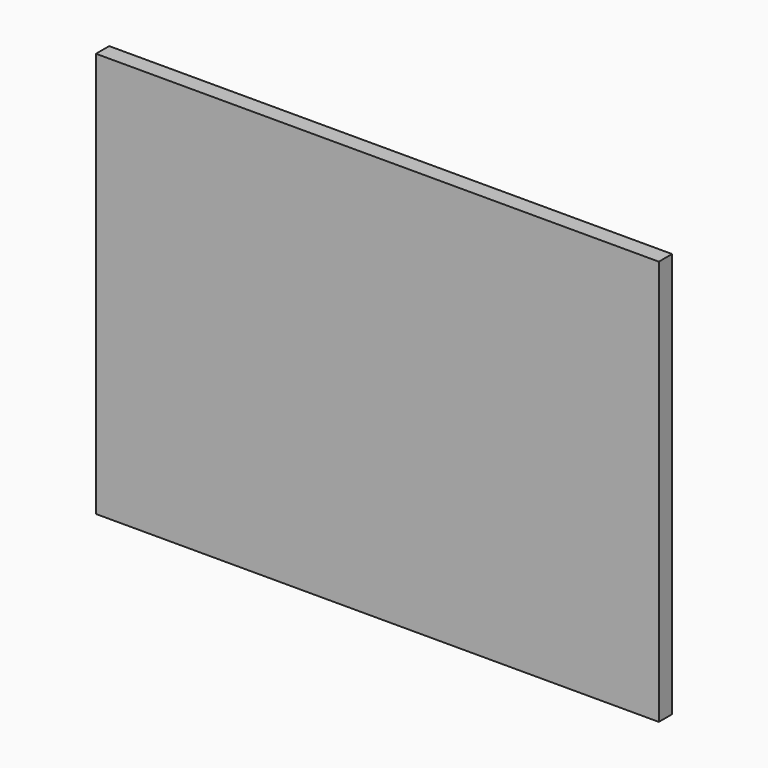
from build123d import *

# Parameters (mm, degrees)
F0_W     = 170
F0_H     = 122.3707973333
F1_DEPTH = 5
F2_R     = 1.5
F3_DEPTH = 5


# Not quite as in the source:
# - a pattern or mirror of a feature is missing from the dataset's text; its kind, count and spacing are read off the source's solid


with BuildPart() as f1:
    # F0 (on Front) → F1 (new body)
    with BuildSketch(Plane.XZ):
        Rectangle(F0_W, F0_H)
    extrude(amount=F1_DEPTH)

    # F2 (on Front) → F3 (join)
    with BuildSketch(Plane.XZ):
        with Locations((70, 56.1853986666)):
            Circle(F2_R)
    f3 = extrude(amount=-F3_DEPTH)

    # F3_copies: F3 across plane
    add(f3.mirror(Plane(origin=(0, 0, 0), x_dir=(0, 0, -1), z_dir=(-1, 0, 0))))

    # F3_copies1: F3 across plane
    add(f3.mirror(Plane(origin=(0, 0, 0), x_dir=(-1, 0, 0), z_dir=(0, 0, -1))))

    # F3_copies2: F3 across plane
    add(f3.mirror(Plane(origin=(0, 0, 0), x_dir=(0.6259536866, 0, -0.7798602325), z_dir=(-0.7798602325, 0, -0.6259536866))))


solid = f1.part
